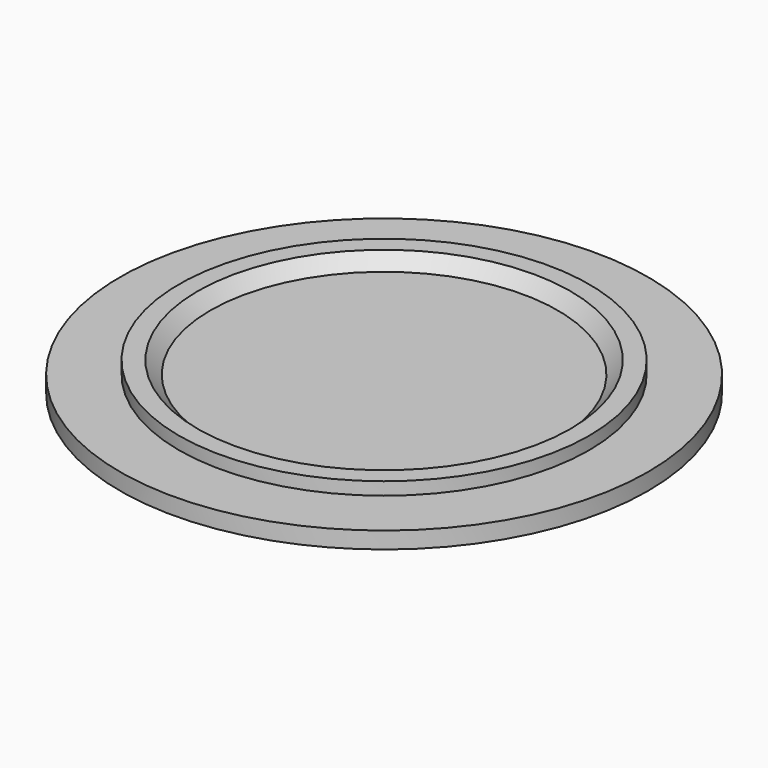
from build123d import *

# Parameters (mm, degrees)
F0_R     = 26.9
F0_R_2   = 20.9
F1_DEPTH = 1.7
F2_DEPTH = 3
F3_R     = 19
F4_DEPTH = 1.3
F5_SIZE  = 1.29999


# Not quite as in the source:
# - a fillet or chamfer is up to 0.001 mm smaller than in the source, because OpenCascade refuses the exact size


with BuildPart() as f1:
    # F0 (on Top) → F1 (new body)
    with BuildSketch(Plane.XY):
        Circle(F0_R)
        Circle(F0_R_2, mode=Mode.SUBTRACT)
    extrude(amount=F1_DEPTH)

    # F0 (on Top) → F2 (join)
    with BuildSketch(Plane.XY):
        Circle(F0_R_2)
    extrude(amount=F2_DEPTH)

    # F3 (on face) → F4 (cut)
    with BuildSketch(Plane.XY.offset(3)):
        Circle(F3_R)
    extrude(amount=-F4_DEPTH, mode=Mode.SUBTRACT)

    # F5 (size 1.3 in the source; OpenCascade refuses exactly that, so slightly less here)
    f5_edges = [f1.edges().sort_by_distance(p)[0] for p in [
        (-19, 0, 1.7),
    ]]
    chamfer(f5_edges, length=F5_SIZE)


solid = f1.part
